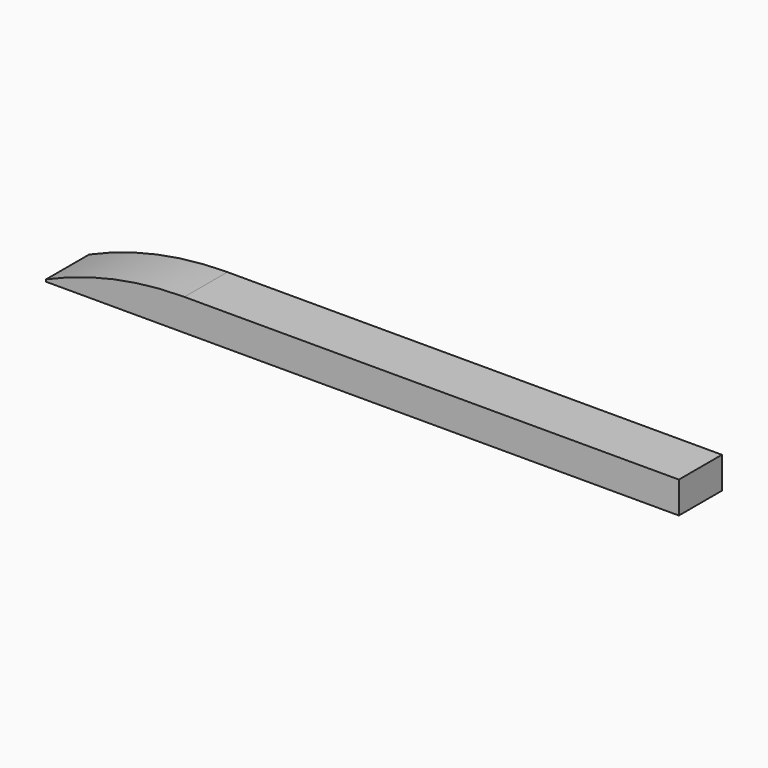
from build123d import *

# Parameters (mm, degrees)
F0_W        = 50
F0_H        = 8.5
F1_DEPTH    = 5
F2_SIZE2    = 4.6630765815
F2_SIZE     = 10
F3_T1_DEPTH = 67.7710723862


# Not quite as in the source:
# - a fillet or chamfer that OpenCascade refuses, or shapes differently, is made with other operations: its cross-section is extruded or revolved along the edge and cut away or added
# - a feature of the source that left no trace in its solid (it failed there, or was rolled back) is left out


with BuildPart() as f1:
    # F0 (on Top) → F1 (new body)
    with BuildSketch(Plane.XY):
        with Locations((-25, 0)):
            Rectangle(F0_W, F0_H)
        with Locations((25, 0)):
            Rectangle(F0_W, F0_H)
    extrude(amount=F1_DEPTH)

    # F2
    f2_edges = [f1.edges().sort_by_distance(p)[0] for p in [
        (-50, 0, 5),
    ]]
    f2_side = f1.faces().sort_by_distance((0, 0, 5))[0]
    chamfer(f2_edges, length=F2_SIZE, length2=F2_SIZE2, reference=f2_side)

    # F3: fillet of radius 53.5430809348 on 1 edges, made by hand

    # F3_s2 → F3_t1 (cut)
    with BuildSketch(Plane.XZ.offset(-33.8855361931)):
        with BuildLine():
            ThreePointArc((-50, 0.3369234184), (-39.3188667185, 3.8212559042), (-28.1457855228, 5))
            Line((-28.1457855228, 5), (-40, 5))
            Line((-40, 5), (-50, 0.3369234184))
        make_face()
    extrude(amount=F3_T1_DEPTH, mode=Mode.SUBTRACT)


solid = f1.part
